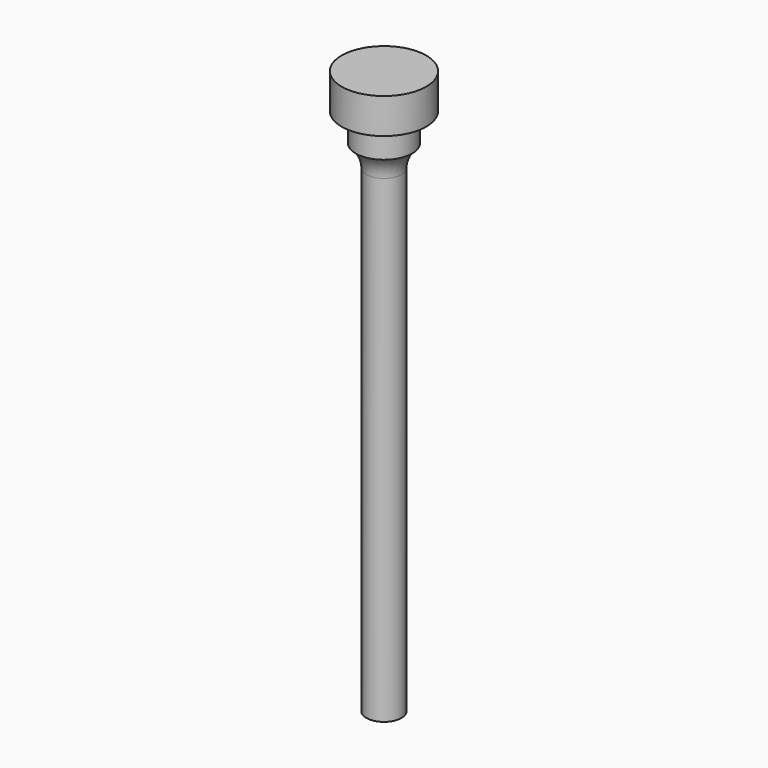
from build123d import *

# Parameters (mm, degrees)
F2_R = 5


# Not quite as in the source:
# - a fillet or chamfer that OpenCascade refuses, or shapes differently, is made with other operations: its cross-section is extruded or revolved along the edge and cut away or added


with BuildPart() as f1:
    # F0 (on Front) → F1 (revolve)
    with BuildSketch(Plane.XZ):
        Polygon((0, -800), (0, 0), (-60, 0), (-60, -50), (-40, -50), (-40, -90), (-25, -90), (-25, -800), align=None)
    revolve(axis=Axis((0, 0, -400), (0, 0, -1)))

    # F2
    f2_edges = [f1.edges().sort_by_distance(p)[0] for p in [
        (40, 0, -50),
    ]]
    fillet(f2_edges, radius=F2_R)

    # F3: fillet of radius 40 on 1 edges, made by hand

    # F3_s1 → F3_t2 (revolve)
    with BuildSketch(Plane.XZ):
        with BuildLine():
            ThreePointArc((-40, -90), (-28.9444872454, -103.9044819163), (-25, -121.224989992))
            Line((-25, -121.224989992), (-25, -90))
            Line((-25, -90), (-40, -90))
        make_face()
    revolve(axis=Axis((0, 0, -90), (0, 0, -1)))


solid = f1.part
